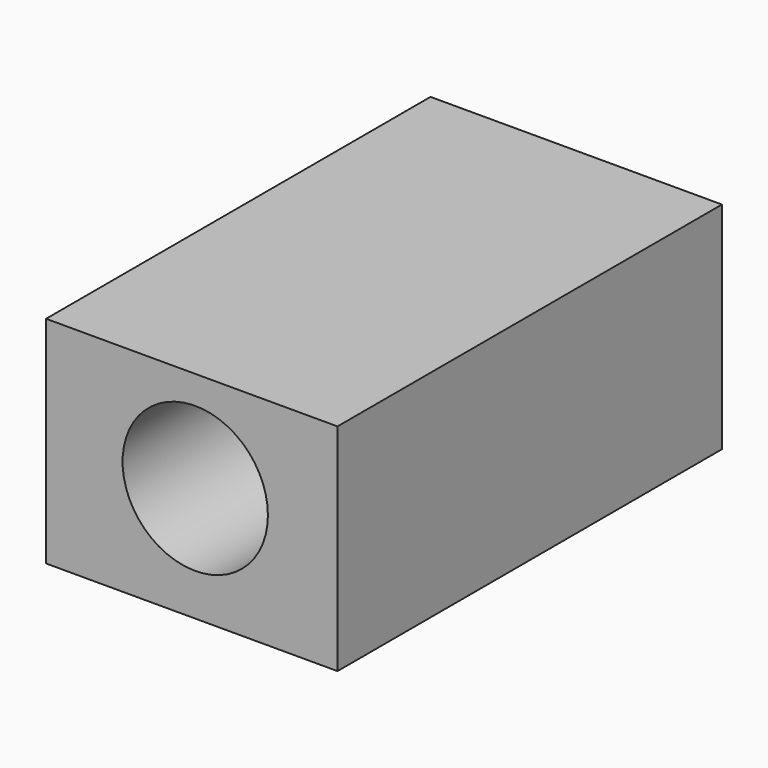
from build123d import *

# Parameters (mm, degrees)
F0_W     = 61.6135448217
F0_H     = 45.5531394109
F0_R     = 15.3630255382
F0_R_2   = 11.4814952194
F1_DEPTH = 50.8
F2_DEPTH = 101.6


# Not quite as in the source:
# - the program builds the solid bodies; features that only make, move or delete a surface that nothing else refers to are left out


with BuildPart() as f1:
    # F0 (on Front) → F1 (new body)
    with BuildSketch(Plane.XZ):
        with Locations((4.0881037712, 8.3222077228)):
            Rectangle(F0_W, F0_H)
        with Locations((4.818121437, 9.7822444513)):
            Circle(F0_R, mode=Mode.SUBTRACT)
        with Locations((4.818121437, 9.7822444513)):
            Circle(F0_R)
        with Locations((4.818121437, 9.7822444513)):
            Circle(F0_R_2, mode=Mode.SUBTRACT)
    extrude(amount=F1_DEPTH)

    # F0 (on Front) → F2 (join)
    with BuildSketch(Plane.XZ):
        with Locations((4.0881037712, 8.3222077228)):
            Rectangle(F0_W, F0_H)
        with Locations((4.818121437, 9.7822444513)):
            Circle(F0_R, mode=Mode.SUBTRACT)
    extrude(amount=F2_DEPTH)


solid = f1.part
